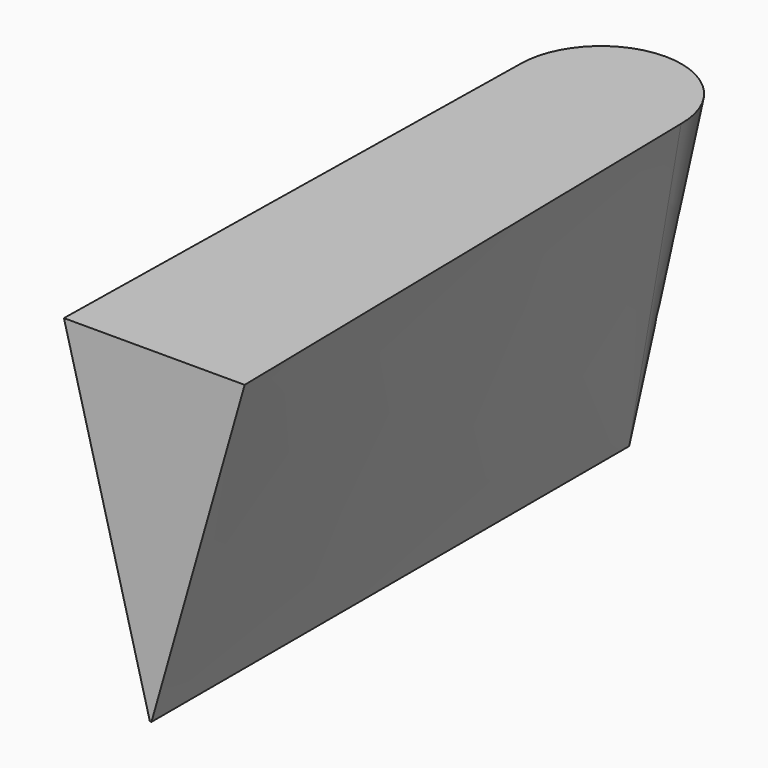
from build123d import *


# Not quite as in the source:
# - ends of sketch curves that miss each other by under 0.0002 mm in the source are joined


with BuildPart() as f3:
    # F1 (on offset) → F3 section 0
    with BuildSketch(Plane.XY.offset(152.4)):
        with BuildLine():
            Line((-42.50436, -194.0035744), (42.50436, -194.0035744))
            Line((42.50436, -194.0035744), (37.9258068, 68.301743))
            ThreePointArc((37.9258068, 68.301743), (0, 106.5075086), (-37.9257970075, 68.301743072))
            Line((-37.9257970075, 68.301743072), (-42.50436, -194.0035744))
        make_face()
    # F2 (on Top) → F3 section 1
    with BuildSketch(Plane.XY):
        with BuildLine():
            Line((-0.3792474, 84.593811), (-0.3792474, -196.1422544))
            Line((-0.3792474, -196.1422544), (0.3792474, -196.1422544))
            Line((0.3792474, -196.1422544), (0.3792474, 84.593811))
            ThreePointArc((0.3792474, 84.593811), (0, 84.9758778), (-0.3792474, 84.593811))
        make_face()
    loft()


solid = f3.part
